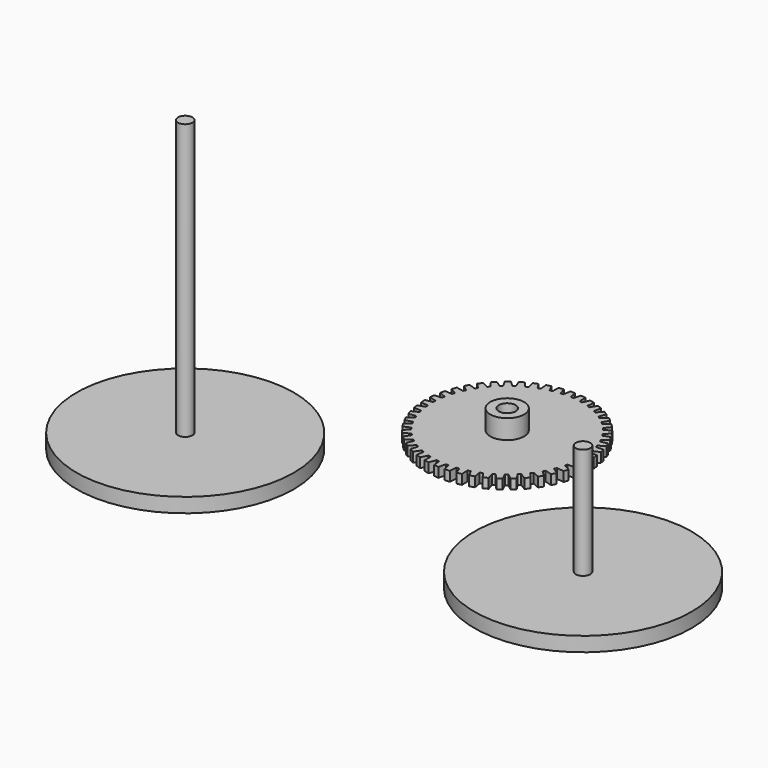
from build123d import *

# Parameters (mm, degrees)
F0_R     = 3.5
F1_DEPTH = 2
F2_DEPTH = 2
F3_COUNT = 47
F0_R_2   = 1.75
F4_DEPTH = 6
F0_R_3   = 1.5
F5_DEPTH = 26
F0_R_4   = 22.5
F6_DEPTH = 3
F7_DEPTH = 60


with BuildPart() as f1:
    # F0 (on Top) → F1 (new body)
    with BuildSketch(Plane.XY):
        with BuildLine():
            ThreePointArc((-0.75, 15.4818442054), (-10.6917023902, -11.2221878437), (15.5, 0))
            ThreePointArc((15.5, 0), (11.2221878437, 10.6917023902), (0.75, 15.4818442054))
            ThreePointArc((0.75, 15.4818442054), (0, 15.5), (-0.75, 15.4818442054))
        make_face()
        Circle(F0_R, mode=Mode.SUBTRACT)
    extrude(amount=F1_DEPTH)

    # F0 (on Top) → F2 (join)
    with BuildSketch(Plane.XY):
        with BuildLine():
            ThreePointArc((-0.75, 15.4818442054), (0, 15.5), (0.75, 15.4818442054))
            Line((0.75, 15.4818442054), (0.5, 16.9818442054))
            Line((0.5, 16.9818442054), (-0.5, 16.9818442054))
            Line((-0.5, 16.9818442054), (-0.75, 15.4818442054))
        make_face()
    extrude(amount=F2_DEPTH)


with BuildPart() as f3_1:
    # F3: instance of F1
    add(f1.part.rotate(Axis((0, 0, 2), (0, 0, -1)), 1 * 360 / F3_COUNT))


with BuildPart() as f3_2:
    # F3: instance of F1
    add(f1.part.rotate(Axis((0, 0, 2), (0, 0, -1)), 2 * 360 / F3_COUNT))


with BuildPart() as f3_3:
    # F3: instance of F1
    add(f1.part.rotate(Axis((0, 0, 2), (0, 0, -1)), 3 * 360 / F3_COUNT))


with BuildPart() as f3_4:
    # F3: instance of F1
    add(f1.part.rotate(Axis((0, 0, 2), (0, 0, -1)), 4 * 360 / F3_COUNT))


with BuildPart() as f3_5:
    # F3: instance of F1
    add(f1.part.rotate(Axis((0, 0, 2), (0, 0, -1)), 5 * 360 / F3_COUNT))


with BuildPart() as f3_6:
    # F3: instance of F1
    add(f1.part.rotate(Axis((0, 0, 2), (0, 0, -1)), 6 * 360 / F3_COUNT))


with BuildPart() as f3_7:
    # F3: instance of F1
    add(f1.part.rotate(Axis((0, 0, 2), (0, 0, -1)), 7 * 360 / F3_COUNT))


with BuildPart() as f3_8:
    # F3: instance of F1
    add(f1.part.rotate(Axis((0, 0, 2), (0, 0, -1)), 8 * 360 / F3_COUNT))


with BuildPart() as f3_9:
    # F3: instance of F1
    add(f1.part.rotate(Axis((0, 0, 2), (0, 0, -1)), 9 * 360 / F3_COUNT))


with BuildPart() as f3_10:
    # F3: instance of F1
    add(f1.part.rotate(Axis((0, 0, 2), (0, 0, -1)), 10 * 360 / F3_COUNT))


with BuildPart() as f3_11:
    # F3: instance of F1
    add(f1.part.rotate(Axis((0, 0, 2), (0, 0, -1)), 11 * 360 / F3_COUNT))


with BuildPart() as f3_12:
    # F3: instance of F1
    add(f1.part.rotate(Axis((0, 0, 2), (0, 0, -1)), 12 * 360 / F3_COUNT))


with BuildPart() as f3_13:
    # F3: instance of F1
    add(f1.part.rotate(Axis((0, 0, 2), (0, 0, -1)), 13 * 360 / F3_COUNT))


with BuildPart() as f3_14:
    # F3: instance of F1
    add(f1.part.rotate(Axis((0, 0, 2), (0, 0, -1)), 14 * 360 / F3_COUNT))


with BuildPart() as f3_15:
    # F3: instance of F1
    add(f1.part.rotate(Axis((0, 0, 2), (0, 0, -1)), 15 * 360 / F3_COUNT))


with BuildPart() as f3_16:
    # F3: instance of F1
    add(f1.part.rotate(Axis((0, 0, 2), (0, 0, -1)), 16 * 360 / F3_COUNT))


with BuildPart() as f3_17:
    # F3: instance of F1
    add(f1.part.rotate(Axis((0, 0, 2), (0, 0, -1)), 17 * 360 / F3_COUNT))


with BuildPart() as f3_18:
    # F3: instance of F1
    add(f1.part.rotate(Axis((0, 0, 2), (0, 0, -1)), 18 * 360 / F3_COUNT))


with BuildPart() as f3_19:
    # F3: instance of F1
    add(f1.part.rotate(Axis((0, 0, 2), (0, 0, -1)), 19 * 360 / F3_COUNT))


with BuildPart() as f3_20:
    # F3: instance of F1
    add(f1.part.rotate(Axis((0, 0, 2), (0, 0, -1)), 20 * 360 / F3_COUNT))


with BuildPart() as f3_21:
    # F3: instance of F1
    add(f1.part.rotate(Axis((0, 0, 2), (0, 0, -1)), 21 * 360 / F3_COUNT))


with BuildPart() as f3_22:
    # F3: instance of F1
    add(f1.part.rotate(Axis((0, 0, 2), (0, 0, -1)), 22 * 360 / F3_COUNT))


with BuildPart() as f3_23:
    # F3: instance of F1
    add(f1.part.rotate(Axis((0, 0, 2), (0, 0, -1)), 23 * 360 / F3_COUNT))


with BuildPart() as f3_24:
    # F3: instance of F1
    add(f1.part.rotate(Axis((0, 0, 2), (0, 0, -1)), 24 * 360 / F3_COUNT))


with BuildPart() as f3_25:
    # F3: instance of F1
    add(f1.part.rotate(Axis((0, 0, 2), (0, 0, -1)), 25 * 360 / F3_COUNT))


with BuildPart() as f3_26:
    # F3: instance of F1
    add(f1.part.rotate(Axis((0, 0, 2), (0, 0, -1)), 26 * 360 / F3_COUNT))


with BuildPart() as f3_27:
    # F3: instance of F1
    add(f1.part.rotate(Axis((0, 0, 2), (0, 0, -1)), 27 * 360 / F3_COUNT))


with BuildPart() as f3_28:
    # F3: instance of F1
    add(f1.part.rotate(Axis((0, 0, 2), (0, 0, -1)), 28 * 360 / F3_COUNT))


with BuildPart() as f3_29:
    # F3: instance of F1
    add(f1.part.rotate(Axis((0, 0, 2), (0, 0, -1)), 29 * 360 / F3_COUNT))


with BuildPart() as f3_30:
    # F3: instance of F1
    add(f1.part.rotate(Axis((0, 0, 2), (0, 0, -1)), 30 * 360 / F3_COUNT))


with BuildPart() as f3_31:
    # F3: instance of F1
    add(f1.part.rotate(Axis((0, 0, 2), (0, 0, -1)), 31 * 360 / F3_COUNT))


with BuildPart() as f3_32:
    # F3: instance of F1
    add(f1.part.rotate(Axis((0, 0, 2), (0, 0, -1)), 32 * 360 / F3_COUNT))


with BuildPart() as f3_33:
    # F3: instance of F1
    add(f1.part.rotate(Axis((0, 0, 2), (0, 0, -1)), 33 * 360 / F3_COUNT))


with BuildPart() as f3_34:
    # F3: instance of F1
    add(f1.part.rotate(Axis((0, 0, 2), (0, 0, -1)), 34 * 360 / F3_COUNT))


with BuildPart() as f3_35:
    # F3: instance of F1
    add(f1.part.rotate(Axis((0, 0, 2), (0, 0, -1)), 35 * 360 / F3_COUNT))


with BuildPart() as f3_36:
    # F3: instance of F1
    add(f1.part.rotate(Axis((0, 0, 2), (0, 0, -1)), 36 * 360 / F3_COUNT))


with BuildPart() as f3_37:
    # F3: instance of F1
    add(f1.part.rotate(Axis((0, 0, 2), (0, 0, -1)), 37 * 360 / F3_COUNT))


with BuildPart() as f3_38:
    # F3: instance of F1
    add(f1.part.rotate(Axis((0, 0, 2), (0, 0, -1)), 38 * 360 / F3_COUNT))


with BuildPart() as f3_39:
    # F3: instance of F1
    add(f1.part.rotate(Axis((0, 0, 2), (0, 0, -1)), 39 * 360 / F3_COUNT))


with BuildPart() as f3_40:
    # F3: instance of F1
    add(f1.part.rotate(Axis((0, 0, 2), (0, 0, -1)), 40 * 360 / F3_COUNT))


with BuildPart() as f3_41:
    # F3: instance of F1
    add(f1.part.rotate(Axis((0, 0, 2), (0, 0, -1)), 41 * 360 / F3_COUNT))


with BuildPart() as f3_42:
    # F3: instance of F1
    add(f1.part.rotate(Axis((0, 0, 2), (0, 0, -1)), 42 * 360 / F3_COUNT))


with BuildPart() as f3_43:
    # F3: instance of F1
    add(f1.part.rotate(Axis((0, 0, 2), (0, 0, -1)), 43 * 360 / F3_COUNT))


with BuildPart() as f3_44:
    # F3: instance of F1
    add(f1.part.rotate(Axis((0, 0, 2), (0, 0, -1)), 44 * 360 / F3_COUNT))


with BuildPart() as f3_45:
    # F3: instance of F1
    add(f1.part.rotate(Axis((0, 0, 2), (0, 0, -1)), 45 * 360 / F3_COUNT))


with BuildPart() as f3_46:
    # F3: instance of F1
    add(f1.part.rotate(Axis((0, 0, 2), (0, 0, -1)), 46 * 360 / F3_COUNT))


with BuildPart() as f1_1:
    add(f1.part)

    add(f3_1.part)  # F4 merges F3_1

    add(f3_2.part)  # F4 merges F3_2

    add(f3_3.part)  # F4 merges F3_3

    add(f3_4.part)  # F4 merges F3_4

    add(f3_5.part)  # F4 merges F3_5

    add(f3_6.part)  # F4 merges F3_6

    add(f3_7.part)  # F4 merges F3_7

    add(f3_8.part)  # F4 merges F3_8

    add(f3_9.part)  # F4 merges F3_9

    add(f3_10.part)  # F4 merges F3_10

    add(f3_11.part)  # F4 merges F3_11

    add(f3_12.part)  # F4 merges F3_12

    add(f3_13.part)  # F4 merges F3_13

    add(f3_14.part)  # F4 merges F3_14

    add(f3_15.part)  # F4 merges F3_15

    add(f3_16.part)  # F4 merges F3_16

    add(f3_17.part)  # F4 merges F3_17

    add(f3_18.part)  # F4 merges F3_18

    add(f3_19.part)  # F4 merges F3_19

    add(f3_20.part)  # F4 merges F3_20

    add(f3_21.part)  # F4 merges F3_21

    add(f3_22.part)  # F4 merges F3_22

    add(f3_23.part)  # F4 merges F3_23

    add(f3_24.part)  # F4 merges F3_24

    add(f3_25.part)  # F4 merges F3_25

    add(f3_26.part)  # F4 merges F3_26

    add(f3_27.part)  # F4 merges F3_27

    add(f3_28.part)  # F4 merges F3_28

    add(f3_29.part)  # F4 merges F3_29

    add(f3_30.part)  # F4 merges F3_30

    add(f3_31.part)  # F4 merges F3_31

    add(f3_32.part)  # F4 merges F3_32

    add(f3_33.part)  # F4 merges F3_33

    add(f3_34.part)  # F4 merges F3_34

    add(f3_35.part)  # F4 merges F3_35

    add(f3_36.part)  # F4 merges F3_36

    add(f3_37.part)  # F4 merges F3_37

    add(f3_38.part)  # F4 merges F3_38

    add(f3_39.part)  # F4 merges F3_39

    add(f3_40.part)  # F4 merges F3_40

    add(f3_41.part)  # F4 merges F3_41

    add(f3_42.part)  # F4 merges F3_42

    add(f3_43.part)  # F4 merges F3_43

    add(f3_44.part)  # F4 merges F3_44

    add(f3_45.part)  # F4 merges F3_45

    add(f3_46.part)  # F4 merges F3_46
    # F0 (on Top) → F4 (join)
    with BuildSketch(Plane.XY):
        Circle(F0_R)
        Circle(F0_R_2, mode=Mode.SUBTRACT)
    extrude(amount=F4_DEPTH)


with BuildPart() as f5:
    # F0 (on Top) → F5 (new body)
    with BuildSketch(Plane.XY):
        with Locations((41.7228154838, -32.5268916786)):
            Circle(F0_R_3)
    extrude(amount=F5_DEPTH)

    # F0 (on Top) → F6 (join)
    with BuildSketch(Plane.XY):
        with Locations((41.7228154838, -32.5268916786)):
            Circle(F0_R_4)
        with Locations((41.7228154838, -32.5268916786)):
            Circle(F0_R_3, mode=Mode.SUBTRACT)
    extrude(amount=F6_DEPTH)


with BuildPart() as f6:
    # F0 (on Top) → F6, piece 2 (new body)
    with BuildSketch(Plane.XY):
        with Locations((-38.9164164662, -34.7063317895)):
            Circle(F0_R_4)
        with Locations((-38.9164164662, -34.7063317895)):
            Circle(F0_R_3, mode=Mode.SUBTRACT)
    extrude(amount=F6_DEPTH)

    # F0 (on Top) → F7 (join)
    with BuildSketch(Plane.XY):
        with Locations((-38.9164164662, -34.7063317895)):
            Circle(F0_R_3)
    extrude(amount=F7_DEPTH)


solid = Compound([f1_1.part, f5.part, f6.part])
